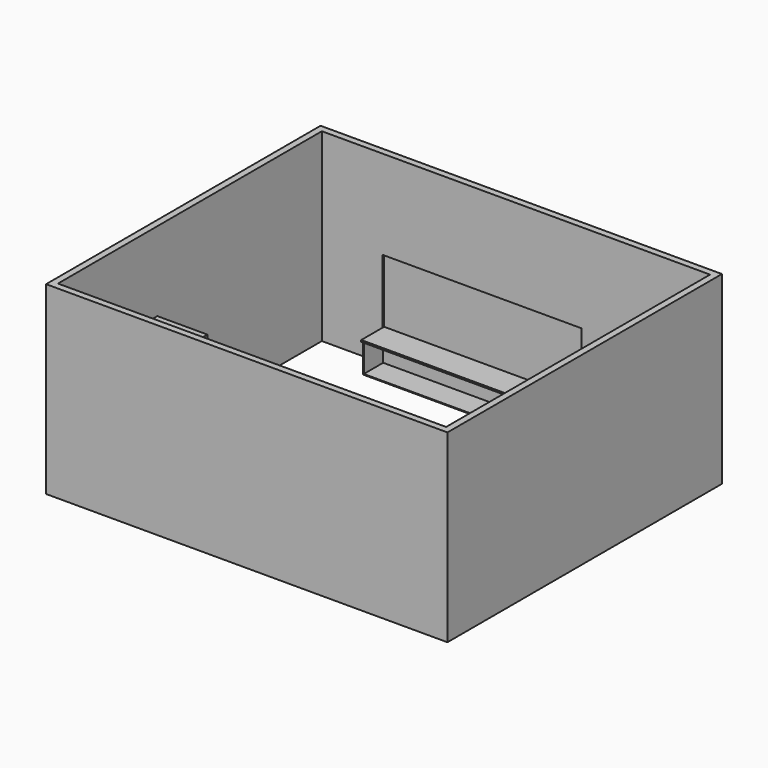
from build123d import *

# Parameters (mm, degrees)
F0_W      = 9271
F0_H      = 7924.8
F1_DEPTH  = 4267.2
F2_DEPTH  = 25.4
F4_W      = 4597.4
F4_H      = 1524
F5_DEPTH  = 152.4
F6_W      = 1003.959779666
F6_H      = 2058.1215861365
F7_DEPTH  = 2438.4
F9_W      = 4597.4
F9_H      = 1524
F10_DEPTH = 25.4
F12_W     = 4597.4
F12_H     = 685.8
F12_W_2   = 4559.3
F12_H_2   = 647.7
F13_DEPTH = 558.8
F11_W     = 4597.4
F11_H     = 38.1
F14_DEPTH = 660.4
F15_W     = 50.8
F15_H     = 50.8
F16_DEPTH = 8966.2


# Not quite as in the source:
# - the program builds the solid bodies; features that only make, move or delete a surface that nothing else refers to are left out


with BuildPart() as f1:
    # F0 (on Top) → F1 (new body)
    with BuildSketch(Plane.XY):
        Rectangle(F0_W, F0_H)
        Polygon((4483.1, 2595.4701114655), (4483.1, -3810), (-4483.1, -3810), (-4483.1, 3810), (2247.9, 3810), (2349.5, 3810), (4483.1, 3810), (4483.1, 2697.0701114655), align=None, mode=Mode.SUBTRACT)
    extrude(amount=F1_DEPTH)

    # F0 (on Top) → F2 (join)
    with BuildSketch(Plane.XY):
        Rectangle(F0_W, F0_H)
        Polygon((4483.1, 2595.4701114655), (4483.1, -3810), (-4483.1, -3810), (-4483.1, 3810), (2247.9, 3810), (2349.5, 3810), (4483.1, 3810), (4483.1, 2697.0701114655), align=None, mode=Mode.SUBTRACT)
    extrude(amount=F2_DEPTH)

    # F4 (on face) → F5 (cut, through all)
    with BuildSketch(Plane(origin=(0, 3962.4, 0), x_dir=(-1, 0, 0), z_dir=(0, 1, 0))):
        with Locations((787.4, 1447.8)):
            Rectangle(F4_W, F4_H)
    extrude(amount=-F5_DEPTH, mode=Mode.SUBTRACT)

    # F6 (on Top) → F7 (join)
    with BuildSketch(Plane.XY):
        Polygon((-3326.740220334, -939.8), (-4483.1, -939.8), (-4483.1, -1092.2), (-3479.140220334, -1092.2), (-3479.140220334, -3150.3215861365), (-4483.1, -3150.3215861365), (-4483.1, -3302.7215861365), (-3326.740220334, -3302.7215861365), align=None)
        with Locations((-3981.120110167, -2121.2607930683)):
            Rectangle(F6_W, F6_H)
    extrude(amount=F7_DEPTH)


with BuildPart() as f10:
    # F9 (on offset) → F10 (new body)
    with BuildSketch(Plane.XZ.offset(-3886.2)):
        with Locations((-787.4, 1447.8)):
            Rectangle(F9_W, F9_H)
    extrude(amount=F10_DEPTH)


with BuildPart() as f13:
    # F12 (on face) → F13 (new body)
    with BuildSketch(Plane.XZ.offset(-3810)):
        with Locations((-787.4, 342.9)):
            Rectangle(F12_W, F12_H)
        with Locations((-787.4, 342.9)):
            Rectangle(F12_W_2, F12_H_2, mode=Mode.SUBTRACT)
    extrude(amount=F13_DEPTH)


with BuildPart() as f14:
    # F11 (on face) → F14 (new body)
    with BuildSketch(Plane.XZ.offset(-3860.8)):
        with Locations((-787.4, 704.85)):
            Rectangle(F11_W, F11_H)
    extrude(amount=F14_DEPTH)


with BuildPart() as f16:
    # F15 (on face) → F16 (new body, through all)
    with BuildSketch(Plane.YZ.offset(-4483.1)):
        with Locations((-914.4, 3276.6)):
            Rectangle(F15_W, F15_H)
    extrude(amount=F16_DEPTH)


solid = Compound([f1.part, f10.part, f13.part, f14.part])
